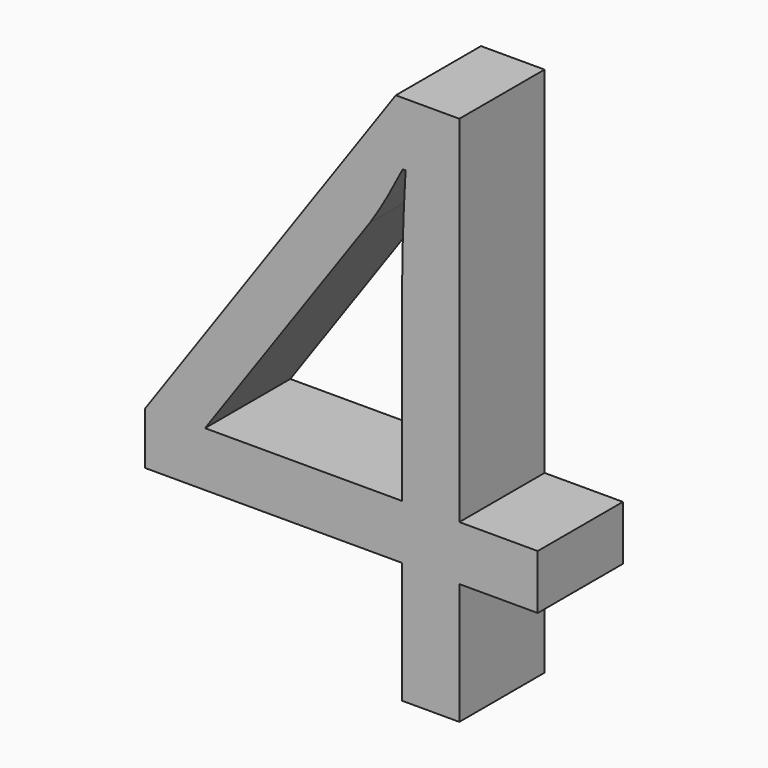
from build123d import *

# Parameters (mm, degrees)
F0_TEXT_SIZE = 35.2777777778
F1_DEPTH     = 5.08


# Not quite as in the source:
# - Text() gives the source's letters only with a copy of the font that has no kerning and outlines rounded to 1/6400 em; it was checked with that copy


with BuildPart() as f1:
    # F0 (on Front) → F1 (new body)
    with BuildSketch(Plane.XZ):
        with Locations((-52.7825179922, 30.9764162362)):
            Text('4', F0_TEXT_SIZE, font='Open Sans', text_align=(TextAlign.LEFT, TextAlign.BOTTOM))
    extrude(amount=F1_DEPTH)


solid = f1.part
